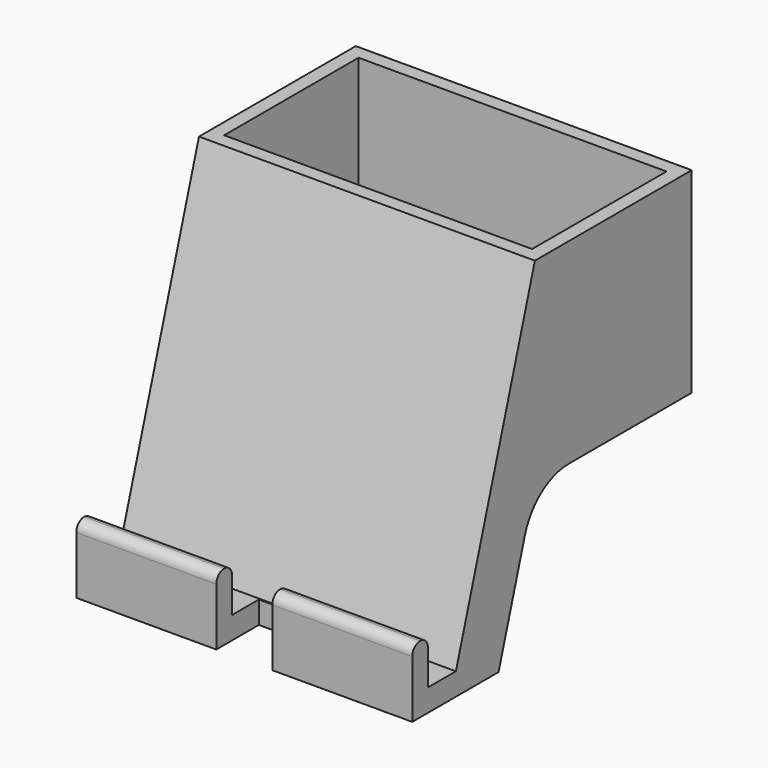
from build123d import *

# Parameters (mm, degrees)
F0_W     = 70
F0_H     = 70
F1_DEPTH = 120
F2_W     = 110
F2_H     = 60
F3_DEPTH = 65
F4_W     = 20
F4_H     = 24.0523201227
F5_DEPTH = 19
F6_R     = 20.5517549394
F7_R     = 3.49999


# Not quite as in the source:
# - a fillet or chamfer is up to 0.001 mm smaller than in the source, because OpenCascade refuses the exact size


with BuildPart() as f1:
    # F0 (on Right) → F1 (new body)
    with BuildSketch(Plane.YZ):
        with Locations((0.0956673622, -2.5781301591)):
            Rectangle(F0_W, F0_H)
        Polygon((-34.9043326378, -37.5781301591), (-34.9043326378, 32.4218698409), (-70.1899622679, -82.3540924191), (-82.6712690592, -82.3540924191), (-82.6712690592, -66.3017722964), (-89.6712690592, -66.3017722964), (-89.6712690592, -82.3540924191), (-89.6712690592, -90.3540924191), (-70.1899622679, -90.3540924191), (-51.1292722594, -90.3540924191), align=None)
    extrude(amount=F1_DEPTH)

    # F2 (on face) → F3 (cut)
    with BuildSketch(Plane.XY.offset(32.4218698409)):
        with Locations((60, 0.0956673622)):
            Rectangle(F2_W, F2_H)
    extrude(amount=-F3_DEPTH, mode=Mode.SUBTRACT)

    # F4 (on face) → F5 (cut)
    with BuildSketch(Plane.XZ.offset(89.6712690592)):
        with Locations((60, -78.3279323578)):
            Rectangle(F4_W, F4_H)
    extrude(amount=-F5_DEPTH, mode=Mode.SUBTRACT)

    # F6
    f6_edges = [f1.edges().sort_by_distance(p)[0] for p in [
        (60, -34.904333, -37.57813),
    ]]
    fillet(f6_edges, radius=F6_R)

    # F7 (radius 3.5 in the source; OpenCascade refuses exactly that, so slightly less here)
    f7_edges = [f1.edges().sort_by_distance(p)[0] for p in [
        (95, -82.671269, -66.301772),
        (25, -82.671269, -66.301772),
        (25, -89.671269, -66.301772),
        (95, -89.671269, -66.301772),
    ]]
    fillet(f7_edges, radius=F7_R)


solid = f1.part
